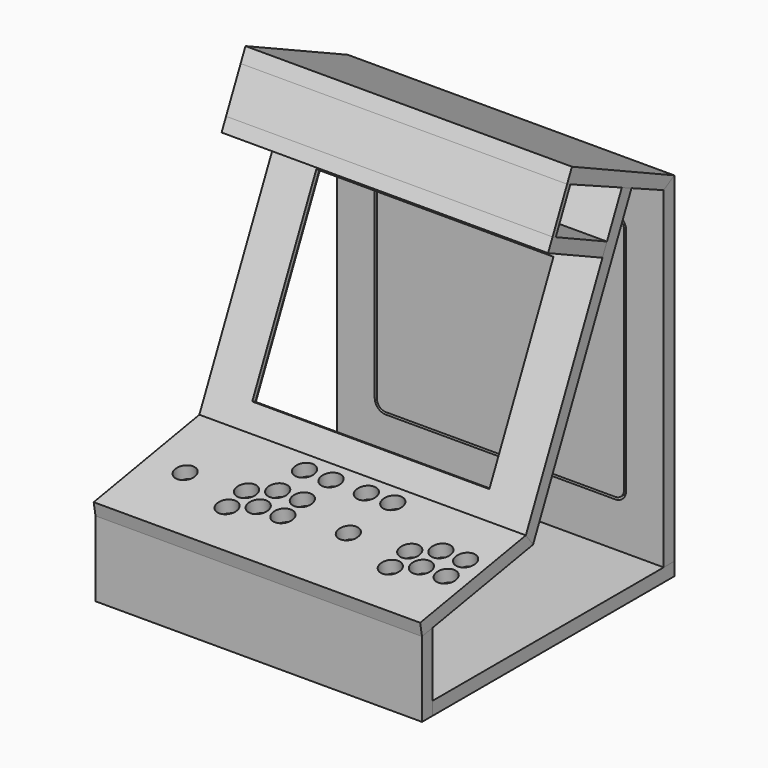
from build123d import *

# Parameters (mm, degrees)
F1_DEPTH  = 469.9
F2_DEPTH  = 469.9
F3_DEPTH  = 469.9
F4_DEPTH  = 469.9
F5_DEPTH  = 469.9
F6_DEPTH  = 469.9
F7_DEPTH  = 469.9
F8_DEPTH  = 469.9
F9_R      = 14.2875
F10_DEPTH = 19.05
F11_W     = 341.3125
F11_H     = 273.05
F12_DEPTH = 19.05
F14_DEPTH = 19.05
F15_W     = 357.1875
F15_H     = 285.75
F15_W_2   = 341.3125
F15_H_2   = 273.05
F16_DEPTH = 12.7


with BuildPart() as f1:
    # F0 (on Right) → F1 (new body)
    with BuildSketch(Plane.YZ):
        Polygon((457.2, 19.05), (457.2, 508), (438.15, 497.0014773719), (438.15, 19.05), align=None)
    extrude(amount=F1_DEPTH)

    # F13 (on face) → F14 (cut)
    with BuildSketch(Plane(origin=(0, 457.2, 0), x_dir=(-1, 0, 0), z_dir=(0, 1, 0))):
        with BuildLine():
            Line((-400.05, 82.55), (-69.85, 82.55))
            ThreePointArc((-69.85, 82.55), (-58.6246798487, 87.1996798487), (-53.975, 98.425))
            Line((-53.975, 98.425), (-53.975, 428.625))
            ThreePointArc((-53.975, 428.625), (-58.6246798487, 439.8503201513), (-69.85, 444.5))
            Line((-69.85, 444.5), (-400.05, 444.5))
            ThreePointArc((-400.05, 444.5), (-411.2753201513, 439.8503201513), (-415.925, 428.625))
            Line((-415.925, 428.625), (-415.925, 98.425))
            ThreePointArc((-415.925, 98.425), (-411.2753201513, 87.1996798487), (-400.05, 82.55))
        make_face()
        with BuildLine():
            Line((-69.85, 85.725), (-400.05, 85.725))
            ThreePointArc((-400.05, 85.725), (-409.0302561211, 89.4447438789), (-412.75, 98.425))
            Line((-412.75, 98.425), (-412.75, 428.625))
            ThreePointArc((-412.75, 428.625), (-409.0302561211, 437.6052561211), (-400.05, 441.325))
            Line((-400.05, 441.325), (-69.85, 441.325))
            ThreePointArc((-69.85, 441.325), (-60.8697438789, 437.6052561211), (-57.15, 428.625))
            Line((-57.15, 428.625), (-57.15, 98.425))
            ThreePointArc((-57.15, 98.425), (-60.8697438789, 89.4447438789), (-69.85, 85.725))
        make_face(mode=Mode.SUBTRACT)
    extrude(amount=-F14_DEPTH, mode=Mode.SUBTRACT)


with BuildPart() as f2:
    # F0 (on Right) → F2 (new body)
    with BuildSketch(Plane.YZ):
        Polygon((438.15, 497.0014773719), (457.2, 508), (273.0382576742, 593.8760307857), (264.3687541785, 575.284220542), (270.1589392144, 572.6759323695), (362.8018997891, 530.94332161), (380.1709667192, 523.1191274677), align=None)
    extrude(amount=F2_DEPTH)


with BuildPart() as f3:
    # F0 (on Right) → F3 (new body)
    with BuildSketch(Plane.YZ):
        Polygon((457.2, 0), (457.2, 19.05), (438.15, 19.05), (22.3579977846, 19.05), (22.3579977846, 0), align=None)
    extrude(amount=F3_DEPTH)


with BuildPart() as f4:
    # F0 (on Right) → F4 (new body)
    with BuildSketch(Plane.YZ):
        Polygon((22.3579977846, 0), (22.3579977846, 19.05), (22.3579977846, 111.5984412876), (3.3079977846, 108.2394123051), (3.3079977846, 0), align=None)
    extrude(amount=F4_DEPTH)


with BuildPart() as f5:
    # F0 (on Right) → F5 (new body)
    with BuildSketch(Plane.YZ):
        Polygon((22.3579977846, 111.5984412876), (203.1400974051, 143.4752030798), (190.067917926, 160.5141020974), (0, 127), (3.3079977846, 108.2394123051), align=None)
    extrude(amount=F5_DEPTH)

    # F9 (on face) → F10 (cut)
    with BuildSketch(Plane(origin=(0, -21.7182791012, 123.1704814199), x_dir=(1, 0, 0), z_dir=(0, -0.1736481777, 0.984807753))):
        with Locations((138.4316366414, 125.5383295276)):
            Circle(F9_R)
        with Locations((138.4316366414, 89.9783295276)):
            Circle(F9_R)
        with Locations((169.2275, 107.7583295276)):
            Circle(F9_R)
        with Locations((169.2275, 143.3183295276)):
            Circle(F9_R)
        with Locations((204.7875, 143.3183295276)):
            Circle(F9_R)
        with Locations((204.7875, 107.7583295276)):
            Circle(F9_R)
        with Locations((171.45, 189.6533404915)):
            Circle(F9_R)
        with Locations((209.55, 189.6533404915)):
            Circle(F9_R)
        with Locations((55.5625, 118.5533295276)):
            Circle(F9_R)
        with Locations((260.35, 189.6533404915)):
            Circle(F9_R)
        with Locations((298.45, 189.6533404915)):
            Circle(F9_R)
        with Locations((290.5125, 118.5533295276)):
            Circle(F9_R)
        with Locations((373.3816366414, 89.9783295276)):
            Circle(F9_R)
        with Locations((373.3816366414, 125.5383295276)):
            Circle(F9_R)
        with Locations((404.1775, 107.7583295276)):
            Circle(F9_R)
        with Locations((404.1775, 143.3183295276)):
            Circle(F9_R)
        with Locations((439.7375, 143.3183295276)):
            Circle(F9_R)
        with Locations((439.7375, 107.7583295276)):
            Circle(F9_R)
    extrude(amount=-F10_DEPTH, mode=Mode.SUBTRACT)


with BuildPart() as f6:
    # F0 (on Right) → F6 (new body)
    with BuildSketch(Plane.YZ):
        Polygon((203.1400974051, 143.4752030798), (380.1709667192, 523.1191274677), (362.8018997891, 530.94332161), (335.9870457781, 473.4386816109), (327.9361678919, 456.1735182679), (190.067917926, 160.5141020974), align=None)
    extrude(amount=F6_DEPTH)

    # F11 (on face) → F12 (cut)
    with BuildSketch(Plane(origin=(0, 94.6401423069, -44.1314231266), x_dir=(1, 0, 0), z_dir=(0, -0.906307787, 0.4226182617))):
        with Locations((234.95, 397.2513537467)):
            Rectangle(F11_W, F11_H)
    extrude(amount=-F12_DEPTH, mode=Mode.SUBTRACT)

    # F15 (on face) → F16 (cut)
    with BuildSketch(Plane(origin=(0, 111.9038265015, -52.1816112745), x_dir=(-1, 0, 0), z_dir=(0, 0.906307787, -0.4226182617))):
        with Locations((-234.95, 397.2513537467)):
            Rectangle(F15_W, F15_H)
        with Locations((-234.95, 397.2513537467)):
            Rectangle(F15_W_2, F15_H_2, mode=Mode.SUBTRACT)
    extrude(amount=-F16_DEPTH, mode=Mode.SUBTRACT)


with BuildPart() as f7:
    # F0 (on Right) → F7 (new body)
    with BuildSketch(Plane.YZ):
        Polygon((243.9061746151, 516.3766970038), (238.1511201675, 519.0603229658), (230.1002422813, 501.7951596228), (327.9361678919, 456.1735182679), (335.9870457781, 473.4386816109), align=None)
    extrude(amount=F7_DEPTH)


with BuildPart() as f8:
    # F0 (on Right) → F8 (new body)
    with BuildSketch(Plane.YZ):
        Polygon((270.1589392144, 572.6759323695), (264.3687541785, 575.284220542), (238.1511201675, 519.0603229658), (243.9061746151, 516.3766970038), align=None)
    extrude(amount=F8_DEPTH)


solid = Compound([f1.part, f2.part, f3.part, f4.part, f5.part, f6.part, f7.part, f8.part])
